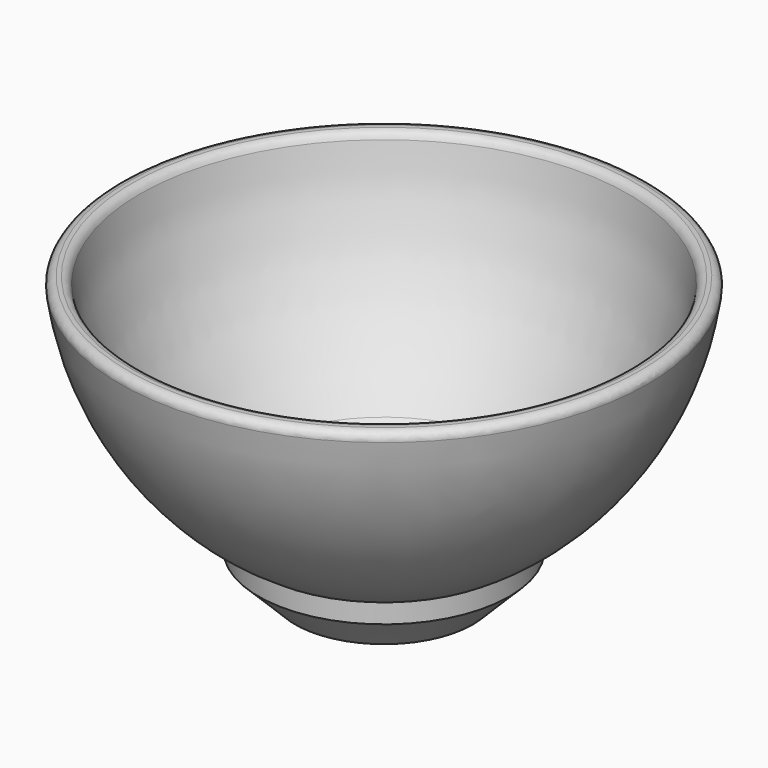
from build123d import *

# Parameters (mm, degrees)
F2_T    = -7.62
F3_SIZE = 13.97
F4_R    = 3.048
F5_R    = 25.4
F6_R    = 5.08


with BuildPart() as f1:
    # F0 (on Front) → F1 (revolve)
    with BuildSketch(Plane.XZ):
        with BuildLine():
            ThreePointArc((48.0706244707, -10.9990021508), (24.9634921318, -21.959563358), (0, -27.5181178004))
            Line((0, -27.5181178004), (0, -32.3714949191))
            Line((0, -32.3714949191), (48.0706244707, -32.3714949191))
            Line((48.0706244707, -32.3714949191), (48.0706244707, -10.9990021508))
        make_face()
        with BuildLine():
            Line((101.6, 74.0818821996), (0, 74.0818821996))
            Line((0, 74.0818821996), (0, -27.5181178004))
            ThreePointArc((0, -27.5181178004), (24.9634921318, -21.959563358), (48.0706244707, -10.9990021508))
            ThreePointArc((48.0706244707, -10.9990021508), (84.6702707915, 25.3536906388), (101.6, 74.0818821996))
        make_face()
    revolve(axis=Axis((0, 0, 23.2818821996), (0, 0, -1)))

    # F2
    f2_openings = [f1.faces().sort_by_distance(p)[0] for p in [
        (0, 0, 74.081882),
    ]]
    offset(amount=F2_T, openings=f2_openings, kind=Kind.INTERSECTION)

    # F3
    f3_edges = [f1.edges().sort_by_distance(p)[0] for p in [
        (-48.070624, 0, -32.371495),
    ]]
    chamfer(f3_edges, length=F3_SIZE)

    # F4
    f4_edges = [f1.edges().sort_by_distance(p)[0] for p in [
        (-101.6, 0, 74.081882),
        (40.450624, 0, -15.754129),
        (-93.932851, 0, 74.081882),
    ]]
    fillet(f4_edges, radius=F4_R)

    # F5
    f5_edges = [f1.edges().sort_by_distance(p)[0] for p in [
        (40.450624, 0, -15.754129),
        (-40.450624, 0.002535, -6.756763),
    ]]
    fillet(f5_edges, radius=F5_R)

    # F6
    f6_edges = [f1.edges().sort_by_distance(p)[0] for p in [
        (-40.450624, 0, -24.751495),
    ]]
    fillet(f6_edges, radius=F6_R)


solid = f1.part
